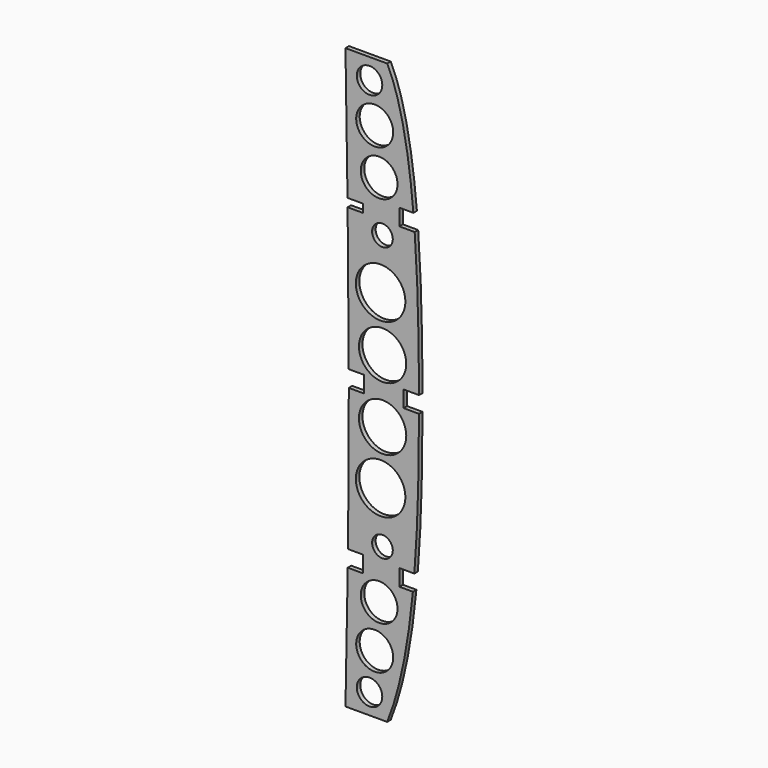
from build123d import *

# Parameters (mm, degrees)
F0_R     = 22.5603447523
F0_R_2   = 21.5516802716
F0_R_3   = 9.418040514
F0_R_4   = 16.7395174503
F0_R_5   = 11.6092445083
F0_R_6   = 16.8526987349
F1_DEPTH = 4


# Not quite as in the source:
# - ends of sketch curves that miss each other by under 0.0002 mm in the source are joined


with BuildPart() as f1:
    # F0 (on Front) → F1 (new body)
    with BuildSketch(Plane.XZ):
        with BuildLine():
            Line((78.8341670899, -6.8383235484), (114.8409428481, -6.8383235484))
            Line((114.8409428481, -6.8383235484), (114.8409428481, 0.6616764516))
            Line((114.8409428481, 0.6616764516), (128.8409428481, 0.6616764516))
            add(Edge.make_bspline(
                [(124.9033857451, 130.1616764516), (127.8407562373, 89.5517987134), (128.7514642032, 44.6895821219), (128.8409428481, 0.6616764516)],
                knots=[0.2778483476, 0.2778483476, 0.2778483476, 0.2778483476, 0.4880499366, 0.4880499366, 0.4880499366, 0.4880499366], degree=3))
            Line((124.9033857451, 130.1616764516), (110.9033857451, 130.1616764516))
            Line((110.9033857451, 130.1616764516), (110.9033857451, 137.6616764516))
            Line((110.9033857451, 137.6616764516), (77.7980855424, 137.6616764516))
            Line((77.7980855424, 137.6616764516), (77.7980855424, 130.1616764516))
            Line((77.7980855424, 130.1616764516), (63.7980855424, 130.1616764516))
            add(Edge.make_bspline(
                [(63.7980855424, 130.1616764516), (64.3462926476, 86.9798084925), (64.7350115683, 43.8051528282), (64.8341670899, 0.6616764516)],
                knots=[0.2404841481, 0.2404841481, 0.2404841481, 0.2404841481, 0.4857851385, 0.4857851385, 0.4857851385, 0.4857851385], degree=3))
            Line((64.8341670899, 0.6616764516), (78.8341670899, 0.6616764516))
            Line((78.8341670899, 0.6616764516), (78.8341670899, -6.8383235484))
        make_face()
        with Locations((93.8518792391, 71.5714693069)):
            Circle(F0_R, mode=Mode.SUBTRACT)
        with Locations((95.6616252661, 22.0235623419)):
            Circle(F0_R_2, mode=Mode.SUBTRACT)
        with Locations((95.5336689949, 117.9889589548)):
            Circle(F0_R_3, mode=Mode.SUBTRACT)
        with BuildLine():
            Line((110.9033857451, 145.1616764516), (123.7062231815, 145.1616764516))
            add(Edge.make_bspline(
                [(99.8484624624, 257.1616764516), (112.2986005896, 232.646487185), (119.5620823416, 192.4052892247), (123.7062231815, 145.1616764516)],
                knots=[0, 0, 0, 0, 0.2516076621, 0.2516076621, 0.2516076621, 0.2516076621], degree=3))
            Line((99.8484624624, 257.1616764516), (61.8484624624, 257.1616764516))
            add(Edge.make_bspline(
                [(61.8484624624, 257.1616764516), (62.5273104324, 217.3359288807), (63.1789559316, 177.4963243829), (63.701293151, 137.6616764516)],
                knots=[0, 0, 0, 0, 0.2262826567, 0.2262826567, 0.2262826567, 0.2262826567], degree=3))
            Line((63.701293151, 137.6616764516), (77.7980855424, 137.6616764516))
            Line((77.7980855424, 137.6616764516), (110.9033857451, 137.6616764516))
            Line((110.9033857451, 137.6616764516), (110.9033857451, 145.1616764516))
        make_face()
        with Locations((92.5064459443, 163.3973568678)):
            Circle(F0_R_4, mode=Mode.SUBTRACT)
        with Locations((83.761125803, 238.4053170681)):
            Circle(F0_R_5, mode=Mode.SUBTRACT)
        with Locations((88.47014606, 203.7603855133)):
            Circle(F0_R_6, mode=Mode.SUBTRACT)
        with BuildLine():
            Line((114.8409428481, -14.3383235484), (114.8409428481, -6.8383235484))
            Line((114.8409428481, -6.8383235484), (78.8341670899, -6.8383235484))
            Line((78.8341670899, -6.8383235484), (78.8341670899, -14.3383235484))
            Line((78.8341670899, -14.3383235484), (64.8568045286, -14.3383235484))
            add(Edge.make_bspline(
                [(64.8568045286, -14.3383235484), (64.8876732357, -57.5094122228), (64.6230490688, -100.6520537776), (64.0989954927, -143.8383235484)],
                knots=[0.51421607, 0.51421607, 0.51421607, 0.51421607, 0.7597151822, 0.7597151822, 0.7597151822, 0.7597151822], degree=3))
            Line((64.0989954927, -143.8383235484), (77.7980855424, -143.8383235484))
            Line((77.7980855424, -143.8383235484), (77.7980855424, -151.3383235484))
            Line((77.7980855424, -151.3383235484), (77.7980855424, -158.8383235484))
            Line((77.7980855424, -158.8383235484), (63.9066232608, -158.8383235484))
            add(Edge.make_bspline(
                [(63.9066232608, -158.8383235484), (63.4029478239, -196.117508426), (62.7091678723, -233.4354001086), (61.8484624624, -270.8383235484)],
                knots=[0.7881349295, 0.7881349295, 0.7881349295, 0.7881349295, 1, 1, 1, 1], degree=3))
            Line((61.8484624624, -270.8383235484), (99.8484624624, -270.8383235484))
            add(Edge.make_bspline(
                [(123.2627847104, -158.8383235484), (119.0509791243, -202.5082607649), (111.8659348538, -240.9997580131), (99.8484624624, -270.8383235484)],
                knots=[0.7571361778, 0.7571361778, 0.7571361778, 0.7571361778, 1, 1, 1, 1], degree=3))
            Line((123.2627847104, -158.8383235484), (110.9033857451, -158.8383235484))
            Line((110.9033857451, -158.8383235484), (110.9033857451, -151.3383235484))
            Line((110.9033857451, -151.3383235484), (110.9033857451, -143.8383235484))
            Line((110.9033857451, -143.8383235484), (124.5795751588, -143.8383235484))
            add(Edge.make_bspline(
                [(128.8408993214, -14.3383234592), (128.7479516437, -59.6820922187), (127.7738982193, -103.6829779906), (124.5795751588, -143.8383235484)],
                knots=[0.5119840968, 0.5119840968, 0.5119840968, 0.5119840968, 0.7296879862, 0.7296879862, 0.7296879862, 0.7296879862], degree=3))
            Line((128.8408993214, -14.3383234592), (114.8409428481, -14.3383235484))
        make_face()
        with Locations((83.761125803, -252.081964165)):
            Circle(F0_R_5, mode=Mode.SUBTRACT)
        with Locations((88.47014606, -217.4370326102)):
            Circle(F0_R_6, mode=Mode.SUBTRACT)
        with Locations((92.5064459443, -177.0740039647)):
            Circle(F0_R_4, mode=Mode.SUBTRACT)
        with Locations((93.8518792391, -85.2481164038)):
            Circle(F0_R, mode=Mode.SUBTRACT)
        with Locations((95.5336689949, -131.6656060517)):
            Circle(F0_R_3, mode=Mode.SUBTRACT)
        with Locations((95.6616252661, -35.7002094388)):
            Circle(F0_R_2, mode=Mode.SUBTRACT)
    extrude(amount=F1_DEPTH)


solid = f1.part
